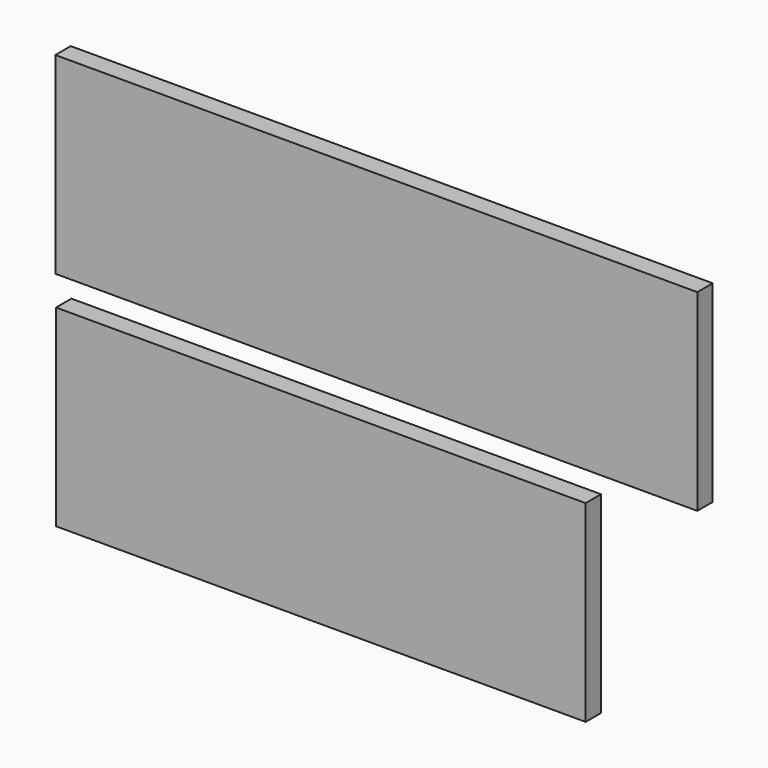
from build123d import *

# Parameters (mm, degrees)
F0_W     = 200
F0_H     = 60
F1_DEPTH = 6
F2_DEPTH = 6
F0_W_2   = 165


# Not quite as in the source:
# - a feature names something its author has since deleted; it is built from what else it names


with BuildPart() as f1:
    # F0 (on Front) → F1 (new body)
    with BuildSketch(Plane.XZ):
        with Locations((42.9789469411, -1.5680367857)):
            Rectangle(F0_W, F0_H)
    extrude(amount=F1_DEPTH)

    # F0 (on Front) → F2 (join)
    with BuildSketch(Plane.XZ):
        with Locations((42.9789469411, -1.5680367857)):
            Rectangle(F0_W, F0_H)
    extrude(amount=F2_DEPTH)


with BuildPart() as f2:
    # F0 (on Front) → F2, piece 2 (new body)
    with BuildSketch(Plane.XZ):
        with Locations((25.7003870606, -70.753903389)):
            Rectangle(F0_W_2, F0_H)
    extrude(amount=F2_DEPTH)


solid = Compound([f1.part, f2.part])
